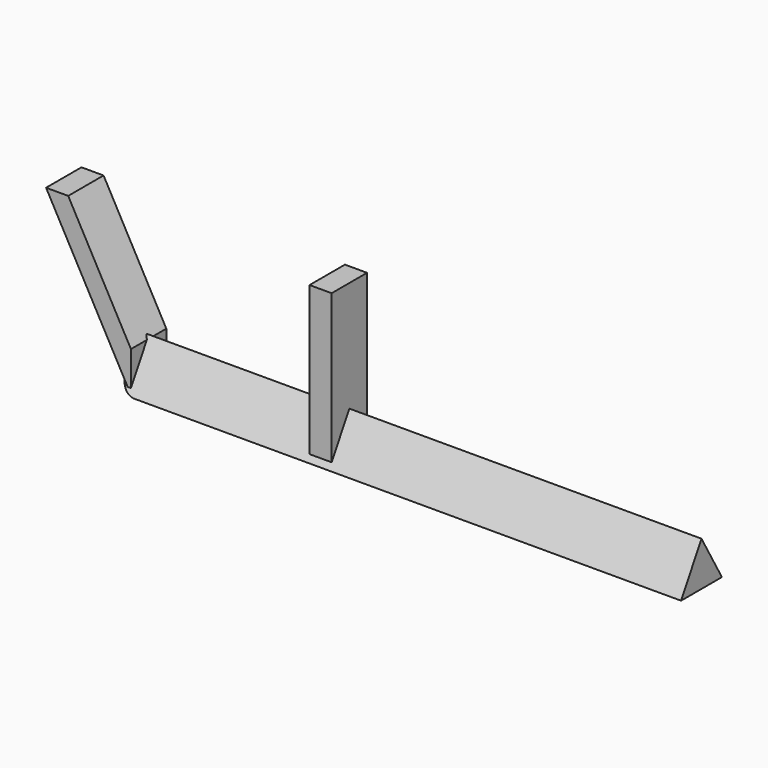
from build123d import *

# Parameters (mm, degrees)
F1_DEPTH      = 63.5
F1_DEPTH_BACK = 1.0668
F2_W          = 2.54
F2_H          = 17.78
F3_DEPTH      = 2.54
F4_DEPTH      = 2.54
F5_R          = 1.77830971


# Not quite as in the source:
# - a feature names something its author has since deleted; it is built from what else it names


with BuildPart() as f1:
    # F0 (on Right) → F1 (new body, two sides)
    with BuildSketch(Plane.YZ) as f1_sk:
        Polygon((2.9329393675, 0), (0, 5.08), (-2.9329393675, 0), align=None)
    extrude(amount=F1_DEPTH)
    extrude(f1_sk.sketch, amount=-F1_DEPTH_BACK)

    # F2 (on Front) → F3 (join, symmetric)
    with BuildSketch(Plane.XZ):
        with Locations((21.7847247761, 8.89)):
            Rectangle(F2_W, F2_H)
    extrude(amount=F3_DEPTH, both=True)

    # F2 (on Front) → F4 (join, symmetric)
    with BuildSketch(Plane.XZ):
        Polygon((-9.746064432, 17.78), (0, 0), (0, 4.6337883681), (-7.206064432, 17.78), align=None)
    extrude(amount=F4_DEPTH, both=True)

    # F5
    f5_edges = [f1.edges().sort_by_distance(p)[0] for p in [
        (-1.0668, 0, 0),
    ]]
    fillet(f5_edges, radius=F5_R)


solid = f1.part
